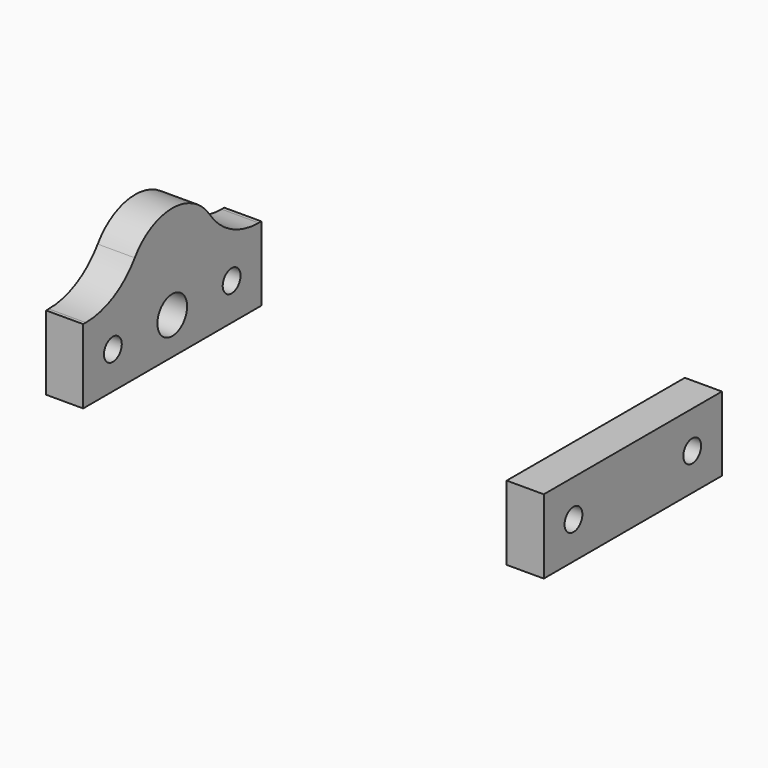
from build123d import *

# Parameters (mm, degrees)
F0_W     = 10
F0_H     = 30
F1_DEPTH = 20
F2_R     = 3
F3_DEPTH = 175
F5_DEPTH = 10
F6_R     = 5
F7_DEPTH = 31.6


with BuildPart() as f1:
    # F0 (on Top) → F1 (new body)
    with BuildSketch(Plane.XY):
        with Locations((-62.0596675936, 15)):
            Rectangle(F0_W, F0_H)
        with Locations((-62.0596675936, -15)):
            Rectangle(F0_W, F0_H)
    extrude(amount=F1_DEPTH)


with BuildPart() as f1b:
    # F0 (on Top) → F1, piece 2 (new body)
    with BuildSketch(Plane.XY):
        Polygon((67.0596675936, 0), (67.0596675936, 30), (57.0596675936, 30), (57.0596675936, 0), (57.0596675936, -30), (67.0596675936, -30), align=None)
    extrude(amount=F1_DEPTH)


with BuildPart() as f3_tool:
    # F2 (on face) → F3 (new body)
    with BuildSketch(Plane.YZ.offset(67.0596675936)):
        with Locations((20, 9.9725276232)):
            Circle(F2_R)
        with Locations((-20, 9.9725276232)):
            Circle(F2_R)
    extrude(amount=-F3_DEPTH)


with BuildPart() as f1_1:
    add(f1.part)

    # F3: cut by f3_tool
    add(f3_tool.part, mode=Mode.SUBTRACT)

    # F4 (on face) → F5 (join, through all)
    with BuildSketch(Plane(origin=(-67.0596675936, 0, 0), x_dir=(0, -1, 0), z_dir=(-1, 0, 0))):
        with BuildLine():
            ThreePointArc((29.0973204207, 20), (19.7854360685, 22.3000336212), (12.6153164249, 28.6711190189))
            ThreePointArc((12.6153164249, 28.6711190189), (0, 35.3079885531), (-12.6153164249, 28.6711190189))
            ThreePointArc((-12.6153164249, 28.6711190189), (-19.7854360685, 22.3000336212), (-29.0973204207, 20))
            Line((-29.0973204207, 20), (29.0973204207, 20))
        make_face()
    extrude(amount=-F5_DEPTH)

    # F6 (on face) → F7 (cut)
    with BuildSketch(Plane(origin=(-67.0596675936, 0, 0), x_dir=(0, -1, 0), z_dir=(-1, 0, 0))):
        with Locations((0, 9.9725276232)):
            Circle(F6_R)
    extrude(amount=-F7_DEPTH, mode=Mode.SUBTRACT)


with BuildPart() as f1b_1:
    add(f1b.part)

    # F3: cut by f3_tool
    add(f3_tool.part, mode=Mode.SUBTRACT)


solid = Compound([f1_1.part, f1b_1.part])
